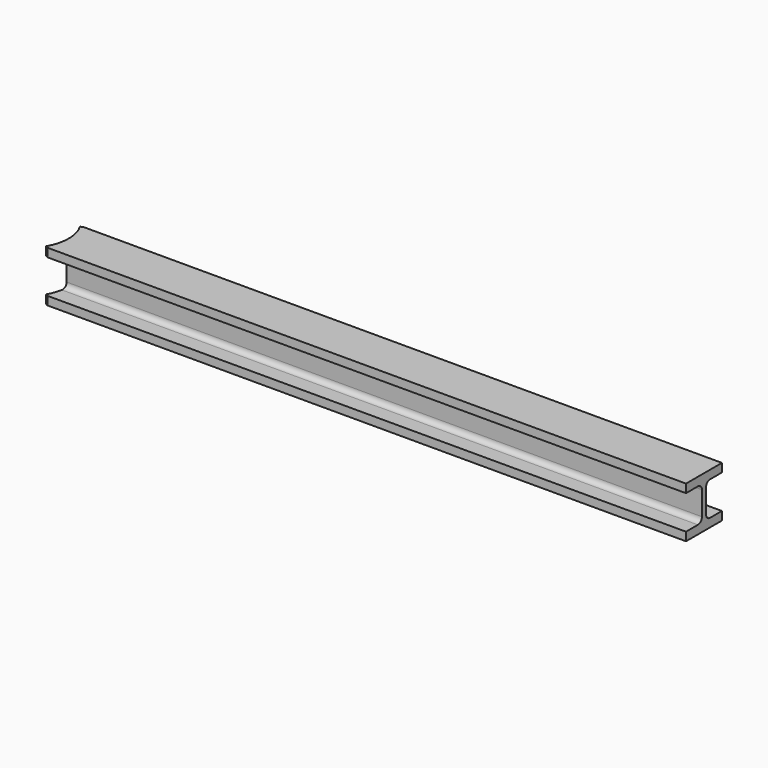
from build123d import *

# Parameters (mm, degrees)
F1_DEPTH     = 20
F3_DEPTH     = 80
F5_DEPTH     = 20
F6_T4_DEPTH  = 1530.1801622923
F6_S5_R      = 100
F6_T6_DEPTH  = 767
F6_T10_DEPTH = 1530.1801622923
F6_S11_R     = 100
F6_T12_DEPTH = 767
F6_T16_DEPTH = 1530.1801622923
F6_S17_R     = 100
F6_T18_DEPTH = 767
F6_T22_DEPTH = 1530.1801622923
F6_S23_R     = 100
F6_T24_DEPTH = 767


# Not quite as in the source:
# - a fillet or chamfer that OpenCascade refuses, or shapes differently, is made with other operations: its cross-section is extruded or revolved along the edge and cut away or added


with BuildPart() as f1:
    # F0 (on Top) → F1 (new body)
    with BuildSketch(Plane.XY):
        with BuildLine():
            Line((1600, -53), (1600, 0))
            Line((1600, 0), (1600, 53))
            Line((1600, 53), (91.7986928012, 53))
            Line((91.7986928012, 53), (86.6025403784, 50))
            ThreePointArc((86.6025403784, 50), (100, 0), (86.6025403784, -50))
            Line((86.6025403784, -50), (91.7986928012, -53))
            Line((91.7986928012, -53), (1600, -53))
        make_face()
    extrude(amount=F1_DEPTH)

    # F2 (on face) → F3 (join)
    with BuildSketch(Plane.XY.offset(20)):
        with BuildLine():
            ThreePointArc((99.8198377077, 6), (100, 0), (99.8198377077, -6))
            Line((99.8198377077, -6), (1600, -6))
            Line((1600, -6), (1600, 6))
            Line((1600, 6), (99.8198377077, 6))
        make_face()
    extrude(amount=F3_DEPTH)

    # F4 (on face) → F5 (join)
    with BuildSketch(Plane.XY.offset(100)):
        with BuildLine():
            ThreePointArc((86.6025403784, 50), (100, 0), (86.6025403784, -50))
            Line((86.6025403784, -50), (91.7986928012, -53))
            Line((91.7986928012, -53), (1600, -53))
            Line((1600, -53), (1600, 53))
            Line((1600, 53), (91.7986928012, 53))
            Line((91.7986928012, 53), (86.6025403784, 50))
        make_face()
    extrude(amount=F5_DEPTH)

    # F6: fillet of radius 12 on 4 edges, made by hand


with BuildPart() as f6_tool2:
    # F6_s3 → F6_t4 (new body)
    with BuildSketch(Plane.YZ.offset(1600)):
        with BuildLine():
            ThreePointArc((6, 32), (9.5147186258, 23.5147186258), (18, 20))
            Line((18, 20), (6, 20))
            Line((6, 20), (6, 32))
        make_face()
    extrude(amount=-F6_T4_DEPTH)

    # F6_s5 → F6_t6 (cut, symmetric)
    with BuildSketch(Plane.XY.offset(26)):
        Circle(F6_S5_R)
    extrude(amount=F6_T6_DEPTH, both=True, mode=Mode.SUBTRACT)


with BuildPart() as f1_1:
    add(f1.part)

    # F6_t1: union F6_tool2
    add(f6_tool2.part)


with BuildPart() as f6_tool8:
    # F6_s9 → F6_t10 (new body)
    with BuildSketch(Plane.YZ.offset(69.8198377077)):
        with BuildLine():
            ThreePointArc((-6, 32), (-9.5147186258, 23.5147186258), (-18, 20))
            Line((-18, 20), (-6, 20))
            Line((-6, 20), (-6, 32))
        make_face()
    extrude(amount=F6_T10_DEPTH)

    # F6_s11 → F6_t12 (cut, symmetric)
    with BuildSketch(Plane.XY.offset(26)):
        Circle(F6_S11_R)
    extrude(amount=F6_T12_DEPTH, both=True, mode=Mode.SUBTRACT)


with BuildPart() as f1_2:
    add(f1_1.part)

    # F6_t7: union F6_tool8
    add(f6_tool8.part)


with BuildPart() as f6_tool14:
    # F6_s15 → F6_t16 (new body)
    with BuildSketch(Plane.YZ.offset(1600)):
        with BuildLine():
            ThreePointArc((18, 100), (9.5147186258, 96.4852813742), (6, 88))
            Line((6, 88), (6, 100))
            Line((6, 100), (18, 100))
        make_face()
    extrude(amount=-F6_T16_DEPTH)

    # F6_s17 → F6_t18 (cut, symmetric)
    with BuildSketch(Plane.XY.offset(94)):
        Circle(F6_S17_R)
    extrude(amount=F6_T18_DEPTH, both=True, mode=Mode.SUBTRACT)


with BuildPart() as f1_3:
    add(f1_2.part)

    # F6_t13: union F6_tool14
    add(f6_tool14.part)


with BuildPart() as f6_tool20:
    # F6_s21 → F6_t22 (new body)
    with BuildSketch(Plane.YZ.offset(69.8198377077)):
        with BuildLine():
            ThreePointArc((-18, 100), (-9.5147186258, 96.4852813742), (-6, 88))
            Line((-6, 88), (-6, 100))
            Line((-6, 100), (-18, 100))
        make_face()
    extrude(amount=F6_T22_DEPTH)

    # F6_s23 → F6_t24 (cut, symmetric)
    with BuildSketch(Plane.XY.offset(94)):
        Circle(F6_S23_R)
    extrude(amount=F6_T24_DEPTH, both=True, mode=Mode.SUBTRACT)


with BuildPart() as f1_4:
    add(f1_3.part)

    # F6_t19: union F6_tool20
    add(f6_tool20.part)


solid = f1_4.part
